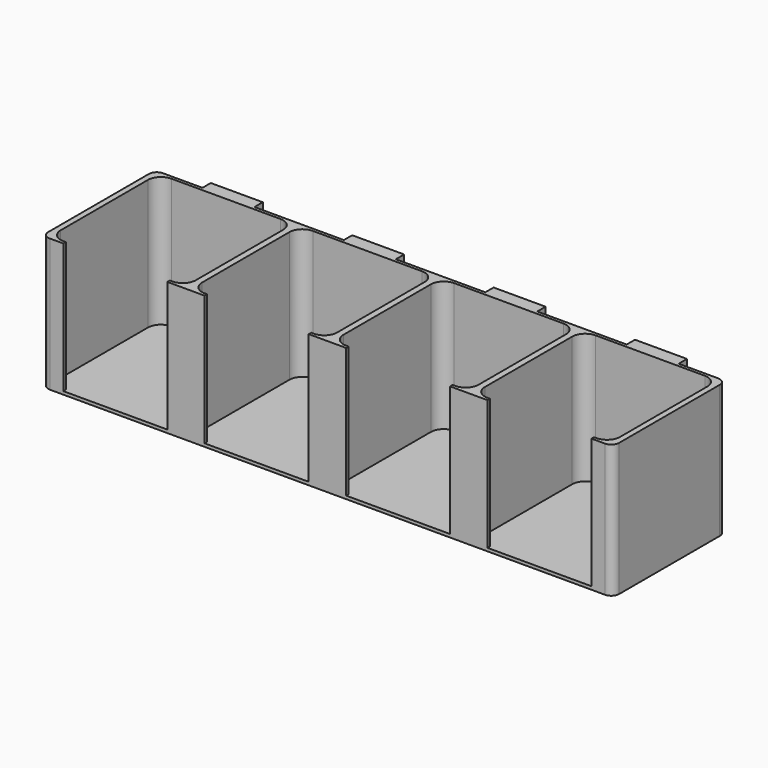
from build123d import *

# Parameters (mm, degrees)
F0_W     = 1
F0_H     = 54.4
F1_DEPTH = 50
F2_W     = 219.6
F2_H     = 54.4
F3_DEPTH = 1.2
F4_W     = 20
F4_H     = 20
F4_R     = 2.5
F5_DEPTH = 5.2
F6_R     = 3
F7_SIZE  = 3.99999


# Not quite as in the source:
# - a fillet or chamfer is up to 0.001 mm smaller than in the source, because OpenCascade refuses the exact size


with BuildPart() as f1:
    # F0 (on Top) → F1 (new body)
    with BuildSketch(Plane.XY):
        with BuildLine():
            Line((-52.5935795337, -9.6814689702), (-53.5935795337, -9.6814689702))
            ThreePointArc((-53.5935795337, -9.6814689702), (-57.1291134396, -8.2170028761), (-58.5935795337, -4.6814689702))
            Line((-58.5935795337, -4.6814689702), (-58.5935795337, 37.3185310298))
            ThreePointArc((-58.5935795337, 37.3185310298), (-57.1291134396, 40.8540649358), (-53.5935795337, 42.3185310298))
            Line((-53.5935795337, 42.3185310298), (-11.5935795337, 42.3185310298))
            ThreePointArc((-11.5935795337, 42.3185310298), (-8.0580456278, 40.8540649358), (-6.5935795337, 37.3185310298))
            Line((-6.5935795337, 37.3185310298), (-6.5935795337, -4.6814689702))
            ThreePointArc((-6.5935795337, -4.6814689702), (-8.0580456278, -8.2170028761), (-11.5935795337, -9.6814689702))
            Line((-11.5935795337, -9.6814689702), (-12.5935795337, -9.6814689702))
            Line((-12.5935795337, -9.6814689702), (-12.5935795337, -10.8814689702))
            Line((-12.5935795337, -10.8814689702), (-5.3935795337, -10.8814689702))
            Line((-5.3935795337, -10.8814689702), (-5.3935795337, 43.5185310298))
            Line((-5.3935795337, 43.5185310298), (-59.7935795337, 43.5185310298))
            Line((-59.7935795337, 43.5185310298), (-59.7935795337, -10.8814689702))
            Line((-59.7935795337, -10.8814689702), (-52.5935795337, -10.8814689702))
            Line((-52.5935795337, -10.8814689702), (-52.5935795337, -9.6814689702))
        make_face()
        with Locations((-60.2935795337, 16.3185310298)):
            Rectangle(F0_W, F0_H)
        with BuildLine():
            Line((49.0064204663, 43.5185310298), (-5.3935795337, 43.5185310298))
            Line((-5.3935795337, 43.5185310298), (-5.3935795337, -10.8814689702))
            Line((-5.3935795337, -10.8814689702), (1.8064204663, -10.8814689702))
            Line((1.8064204663, -10.8814689702), (1.8064204663, -9.6814689702))
            Line((1.8064204663, -9.6814689702), (0.8064204663, -9.6814689702))
            ThreePointArc((0.8064204663, -9.6814689702), (-2.7291134396, -8.2170028761), (-4.1935795337, -4.6814689702))
            Line((-4.1935795337, -4.6814689702), (-4.1935795337, 37.3185310298))
            ThreePointArc((-4.1935795337, 37.3185310298), (-2.7291134396, 40.8540649358), (0.8064204663, 42.3185310298))
            Line((0.8064204663, 42.3185310298), (42.8064204663, 42.3185310298))
            ThreePointArc((42.8064204663, 42.3185310298), (46.3419543722, 40.8540649358), (47.8064204663, 37.3185310298))
            Line((47.8064204663, 37.3185310298), (47.8064204663, -4.6814689702))
            ThreePointArc((47.8064204663, -4.6814689702), (46.3419543722, -8.2170028761), (42.8064204663, -9.6814689702))
            Line((42.8064204663, -9.6814689702), (41.8064204663, -9.6814689702))
            Line((41.8064204663, -9.6814689702), (41.8064204663, -10.8814689702))
            Line((41.8064204663, -10.8814689702), (49.0064204663, -10.8814689702))
            Line((49.0064204663, -10.8814689702), (49.0064204663, 43.5185310298))
        make_face()
        with BuildLine():
            Line((103.4064204663, 43.5185310298), (49.0064204663, 43.5185310298))
            Line((49.0064204663, 43.5185310298), (49.0064204663, -10.8814689702))
            Line((49.0064204663, -10.8814689702), (56.2064204663, -10.8814689702))
            Line((56.2064204663, -10.8814689702), (56.2064204663, -9.6814689702))
            Line((56.2064204663, -9.6814689702), (55.2064204663, -9.6814689702))
            ThreePointArc((55.2064204663, -9.6814689702), (51.6708865604, -8.2170028761), (50.2064204663, -4.6814689702))
            Line((50.2064204663, -4.6814689702), (50.2064204663, 37.3185310298))
            ThreePointArc((50.2064204663, 37.3185310298), (51.6708865604, 40.8540649358), (55.2064204663, 42.3185310298))
            Line((55.2064204663, 42.3185310298), (97.2064204663, 42.3185310298))
            ThreePointArc((97.2064204663, 42.3185310298), (100.7419543722, 40.8540649358), (102.2064204663, 37.3185310298))
            Line((102.2064204663, 37.3185310298), (102.2064204663, -4.6814689702))
            ThreePointArc((102.2064204663, -4.6814689702), (100.7419543722, -8.2170028761), (97.2064204663, -9.6814689702))
            Line((97.2064204663, -9.6814689702), (96.2064204663, -9.6814689702))
            Line((96.2064204663, -9.6814689702), (96.2064204663, -10.8814689702))
            Line((96.2064204663, -10.8814689702), (103.4064204663, -10.8814689702))
            Line((103.4064204663, -10.8814689702), (103.4064204663, 43.5185310298))
        make_face()
        with BuildLine():
            Line((157.8064204663, 43.5185310298), (103.4064204663, 43.5185310298))
            Line((103.4064204663, 43.5185310298), (103.4064204663, -10.8814689702))
            Line((103.4064204663, -10.8814689702), (110.6064204663, -10.8814689702))
            Line((110.6064204663, -10.8814689702), (110.6064204663, -9.6814689702))
            Line((110.6064204663, -9.6814689702), (109.6064204663, -9.6814689702))
            ThreePointArc((109.6064204663, -9.6814689702), (106.0708865604, -8.2170028761), (104.6064204663, -4.6814689702))
            Line((104.6064204663, -4.6814689702), (104.6064204663, 37.3185310298))
            ThreePointArc((104.6064204663, 37.3185310298), (106.0708865604, 40.8540649358), (109.6064204663, 42.3185310298))
            Line((109.6064204663, 42.3185310298), (151.6064204663, 42.3185310298))
            ThreePointArc((151.6064204663, 42.3185310298), (155.1419543722, 40.8540649358), (156.6064204663, 37.3185310298))
            Line((156.6064204663, 37.3185310298), (156.6064204663, -4.6814689702))
            ThreePointArc((156.6064204663, -4.6814689702), (155.1419543722, -8.2170028761), (151.6064204663, -9.6814689702))
            Line((151.6064204663, -9.6814689702), (150.6064204663, -9.6814689702))
            Line((150.6064204663, -9.6814689702), (150.6064204663, -10.8814689702))
            Line((150.6064204663, -10.8814689702), (157.8064204663, -10.8814689702))
            Line((157.8064204663, -10.8814689702), (157.8064204663, 43.5185310298))
        make_face()
        with Locations((158.3064204663, 16.3185310298)):
            Rectangle(F0_W, F0_H)
    extrude(amount=F1_DEPTH)

    # F2 (on face) → F3 (join)
    with BuildSketch(Plane(origin=(0, 0, 0), x_dir=(1, 0, 0), z_dir=(0, 0, -1))):
        with Locations((49.0064204663, -16.3185310298)):
            Rectangle(F2_W, F2_H)
    extrude(amount=F3_DEPTH)

    # F4 (on face) → F5 (join)
    with BuildSketch(Plane.XZ.offset(-42.3185310298)):
        with Locations((-32.5935795337, 40)):
            Rectangle(F4_W, F4_H)
        with Locations((-38.5935795337, 34)):
            Circle(F4_R, mode=Mode.SUBTRACT)
        with Locations((-32.5935795337, 34)):
            Circle(F4_R, mode=Mode.SUBTRACT)
        with Locations((-26.5935795337, 34)):
            Circle(F4_R, mode=Mode.SUBTRACT)
        with Locations((-38.5935795337, 40)):
            Circle(F4_R, mode=Mode.SUBTRACT)
        with Locations((-32.5935795337, 40)):
            Circle(F4_R, mode=Mode.SUBTRACT)
        with Locations((-26.5935795337, 40)):
            Circle(F4_R, mode=Mode.SUBTRACT)
        with Locations((-38.5935795337, 46)):
            Circle(F4_R, mode=Mode.SUBTRACT)
        with Locations((-32.5935795337, 46)):
            Circle(F4_R, mode=Mode.SUBTRACT)
        with Locations((-26.5935795337, 46)):
            Circle(F4_R, mode=Mode.SUBTRACT)
        with Locations((21.8064204663, 40)):
            Rectangle(F4_W, F4_H)
        with Locations((15.8064204663, 34)):
            Circle(F4_R, mode=Mode.SUBTRACT)
        with Locations((21.8064204663, 34)):
            Circle(F4_R, mode=Mode.SUBTRACT)
        with Locations((27.8064204663, 34)):
            Circle(F4_R, mode=Mode.SUBTRACT)
        with Locations((15.8064204663, 40)):
            Circle(F4_R, mode=Mode.SUBTRACT)
        with Locations((21.8064204663, 40)):
            Circle(F4_R, mode=Mode.SUBTRACT)
        with Locations((27.8064204663, 40)):
            Circle(F4_R, mode=Mode.SUBTRACT)
        with Locations((15.8064204663, 46)):
            Circle(F4_R, mode=Mode.SUBTRACT)
        with Locations((21.8064204663, 46)):
            Circle(F4_R, mode=Mode.SUBTRACT)
        with Locations((27.8064204663, 46)):
            Circle(F4_R, mode=Mode.SUBTRACT)
        with Locations((76.2064204663, 40)):
            Rectangle(F4_W, F4_H)
        with Locations((70.2064204663, 34)):
            Circle(F4_R, mode=Mode.SUBTRACT)
        with Locations((76.2064204663, 34)):
            Circle(F4_R, mode=Mode.SUBTRACT)
        with Locations((82.2064204663, 34)):
            Circle(F4_R, mode=Mode.SUBTRACT)
        with Locations((70.2064204663, 40)):
            Circle(F4_R, mode=Mode.SUBTRACT)
        with Locations((76.2064204663, 40)):
            Circle(F4_R, mode=Mode.SUBTRACT)
        with Locations((82.2064204663, 40)):
            Circle(F4_R, mode=Mode.SUBTRACT)
        with Locations((70.2064204663, 46)):
            Circle(F4_R, mode=Mode.SUBTRACT)
        with Locations((76.2064204663, 46)):
            Circle(F4_R, mode=Mode.SUBTRACT)
        with Locations((82.2064204663, 46)):
            Circle(F4_R, mode=Mode.SUBTRACT)
        with Locations((130.6064204663, 40)):
            Rectangle(F4_W, F4_H)
        with Locations((124.6064204663, 34)):
            Circle(F4_R, mode=Mode.SUBTRACT)
        with Locations((130.6064204663, 34)):
            Circle(F4_R, mode=Mode.SUBTRACT)
        with Locations((136.6064204663, 34)):
            Circle(F4_R, mode=Mode.SUBTRACT)
        with Locations((124.6064204663, 40)):
            Circle(F4_R, mode=Mode.SUBTRACT)
        with Locations((130.6064204663, 40)):
            Circle(F4_R, mode=Mode.SUBTRACT)
        with Locations((136.6064204663, 40)):
            Circle(F4_R, mode=Mode.SUBTRACT)
        with Locations((124.6064204663, 46)):
            Circle(F4_R, mode=Mode.SUBTRACT)
        with Locations((130.6064204663, 46)):
            Circle(F4_R, mode=Mode.SUBTRACT)
        with Locations((136.6064204663, 46)):
            Circle(F4_R, mode=Mode.SUBTRACT)
    extrude(amount=-F5_DEPTH)

    # F6
    f6_edges = [f1.edges().sort_by_distance(p)[0] for p in [
        (-60.79358, -10.881469, 24.4),
        (158.80642, -10.881469, 24.4),
        (-60.79358, 43.518531, 24.4),
        (158.80642, 43.518531, 24.4),
    ]]
    fillet(f6_edges, radius=F6_R)

    # F7 (size 4 in the source; OpenCascade refuses exactly that, so slightly less here)
    f7_edges = [f1.edges().sort_by_distance(p)[0] for p in [
        (130.60642, 43.518531, 30),
        (76.20642, 43.518531, 30),
        (21.80642, 43.518531, 30),
        (-32.59358, 43.518531, 30),
    ]]
    chamfer(f7_edges, length=F7_SIZE)


solid = f1.part
